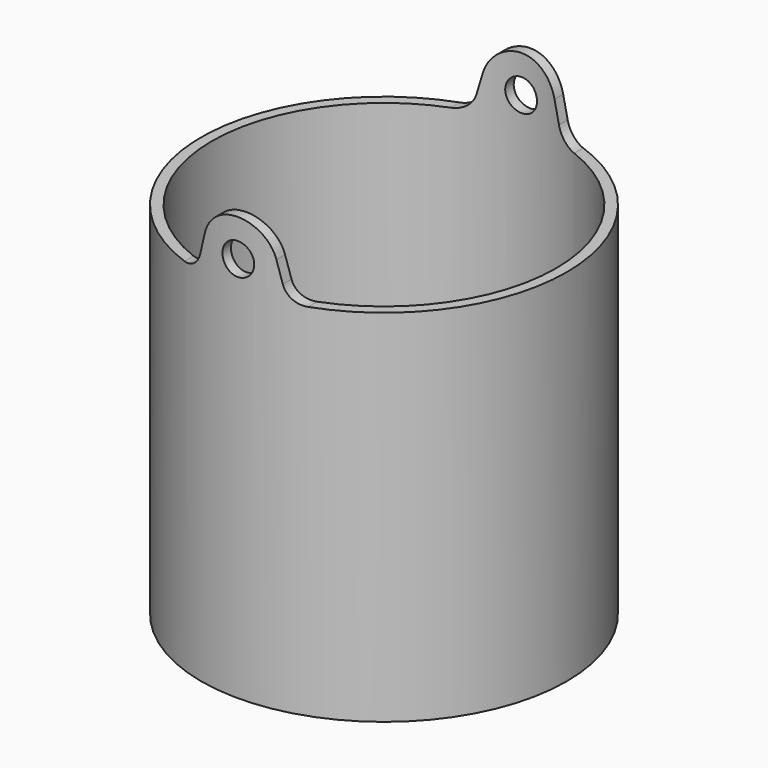
from build123d import *

# Parameters (mm, degrees)
F1_R     = 43.815
F1_R_2   = 41.275
F2_DEPTH = 101.6
F3_DEPTH = 2.54
F4_R     = 3.81
F5_DEPTH = 57.658
F6_R     = 5.08


# Not quite as in the source:
# - a variable given as a bare number and used for a length is read in inches; the dataset says mm whatever the document's units were


with BuildPart() as f2:
    # F1 (on Top) → F2 (new body)
    with BuildSketch(Plane.XY):
        Circle(F1_R)
        Circle(F1_R_2, mode=Mode.SUBTRACT)
    extrude(amount=F2_DEPTH)

    # F1 (on Top) → F3 (join)
    with BuildSketch(Plane.XY):
        Circle(F1_R_2)
    extrude(amount=F3_DEPTH)

    # F4 (on Front) → F5 (cut, symmetric)
    with BuildSketch(Plane.XZ):
        with Locations((0, 92.71)):
            Circle(F4_R)
        with BuildLine():
            Line((46.664010312, 104.1751918972), (-46.664010312, 104.1751918972))
            Line((-46.664010312, 104.1751918972), (-46.664010312, 86.36))
            Line((-46.664010312, 86.36), (-10.9050826158, 86.36))
            Line((-10.9050826158, 86.36), (-8.5870805957, 95.010901311))
            ThreePointArc((-8.5870805957, 95.010901311), (0, 101.6), (8.5870805957, 95.010901311))
            Line((8.5870805957, 95.010901311), (10.9050826158, 86.36))
            Line((10.9050826158, 86.36), (46.664010312, 86.36))
            Line((46.664010312, 86.36), (46.664010312, 104.1751918972))
        make_face()
    extrude(amount=F5_DEPTH, both=True, mode=Mode.SUBTRACT)

    # F6
    f6_edges = [f2.edges().sort_by_distance(p)[0] for p in [
        (10.905083, -41.122289, 86.36),
        (10.905083, 41.122289, 86.36),
        (-10.905083, -41.122289, 86.36),
        (-10.905083, 41.122289, 86.36),
    ]]
    fillet(f6_edges, radius=F6_R)


solid = f2.part
